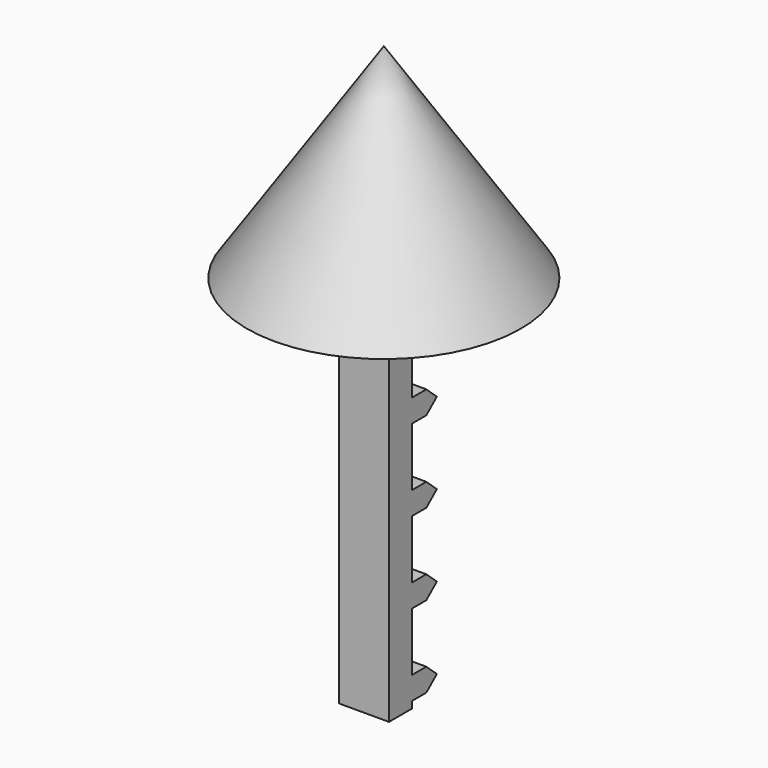
from build123d import *

# Parameters (mm, degrees)
F3_W      = 12.7
F3_H      = 12.7
F4_DEPTH  = 78.486
F6_DEPTH  = 56.134
F8_DEPTH  = 25.4
F10_DEPTH = 25.4


# Not quite as in the source:
# - a feature names something its author has since deleted; it is built from what else it names


with BuildPart() as f1:
    # F0 (on Right) → F1 (revolve)
    with BuildSketch(Plane.YZ):
        Polygon((0, 43.3274172246), (-29.0957745165, 0), (0, 0), align=None)
    revolve(axis=Axis((0, 0, 21.6637086123), (0, 0, -1)))

    # F3 (on face) → F4 (join)
    with BuildSketch(Plane(origin=(0, 0, 0), x_dir=(1, 0, 0), z_dir=(0, 0, -1))):
        with Locations((-0.3540940419, -0.2081472591)):
            Rectangle(F3_W, F3_H)
    extrude(amount=F4_DEPTH)

    # F5 (on face) → F6 (join)
    with BuildSketch(Plane.YZ.offset(5.9959059581)):
        Polygon((0, -7.9661617056), (0, -3.1097470783), (0, 0), (-6.1418527409, 0), (-6.1418527409, -78.486), (0, -78.486), (0, -77.0541617056), (0, -72.1977470783), (0, -59.7821617056), (0, -54.9257470783), (0, -42.5101617056), (0, -37.6537470783), (0, -25.2381617056), (0, -20.3817470783), align=None)
        Polygon((3.7682792172, -3.1097470783), (0, -3.1097470783), (0, -7.9661617056), (3.7682792172, -7.9661617056), (6.5581472591, -5.6115360931), align=None)
        Polygon((3.7682792172, -20.3817470783), (0, -20.3817470783), (0, -25.2381617056), (3.7682792172, -25.2381617056), (6.5581472591, -22.8835360931), align=None)
        Polygon((3.7682792172, -42.5101617056), (6.5581472591, -40.1555360931), (3.7682792172, -37.6537470783), (0, -37.6537470783), (0, -42.5101617056), align=None)
        Polygon((3.7682792172, -59.7821617056), (6.5581472591, -57.4275360931), (3.7682792172, -54.9257470783), (0, -54.9257470783), (0, -59.7821617056), align=None)
        Polygon((0, -72.1977470783), (0, -77.0541617056), (3.7682792172, -77.0541617056), (6.5581472591, -74.6995360931), (3.7682792172, -72.1977470783), align=None)
    extrude(amount=-F6_DEPTH)

    # F5 (on face) → F8 (cut)
    with BuildSketch(Plane.YZ.offset(5.9959059581)):
        Polygon((0, 0), (0, -3.1097470783), (3.7682792172, -3.1097470783), (6.5581472591, -5.6115360931), (6.5581472591, 0), align=None)
        Polygon((3.7682792172, -7.9661617056), (0, -7.9661617056), (0, -20.3817470783), (3.7682792172, -20.3817470783), (6.5581472591, -22.8835360931), (6.5581472591, -5.6115360931), align=None)
        Polygon((6.5581472591, -40.1555360931), (6.5581472591, -22.8835360931), (3.7682792172, -25.2381617056), (0, -25.2381617056), (0, -37.6537470783), (3.7682792172, -37.6537470783), align=None)
        Polygon((6.5581472591, -57.4275360931), (6.5581472591, -40.1555360931), (3.7682792172, -42.5101617056), (0, -42.5101617056), (0, -54.9257470783), (3.7682792172, -54.9257470783), align=None)
        Polygon((6.5581472591, -74.6995360931), (6.5581472591, -57.4275360931), (3.7682792172, -59.7821617056), (0, -59.7821617056), (0, -72.1977470783), (3.7682792172, -72.1977470783), align=None)
        Polygon((0, -77.0541617056), (0, -78.486), (6.5581472591, -78.486), (6.5581472591, -74.6995360931), (3.7682792172, -77.0541617056), align=None)
    extrude(amount=-F8_DEPTH, mode=Mode.SUBTRACT)

    # F9 (on face) → F10 (cut)
    with BuildSketch(Plane.XZ.offset(6.1418527409)):
        Polygon((-4.6626133844, -78.486), (-4.6626133844, 0), (-28.4401431013, 0), (-50.1380940419, 0), (-50.1380940419, -78.486), align=None)
    extrude(amount=-F10_DEPTH, mode=Mode.SUBTRACT)


with BuildPart() as f2:
    # F0 (on Right) → F2 (revolve)
    with BuildSketch(Plane.YZ):
        Polygon((122.2083866596, 0), (151.3041611761, 0), (122.2083866596, 43.3274172246), align=None)
    revolve(axis=Axis((0, 122.2083866596, 21.6637086123), (0, 0, -1)))


solid = f1.part
